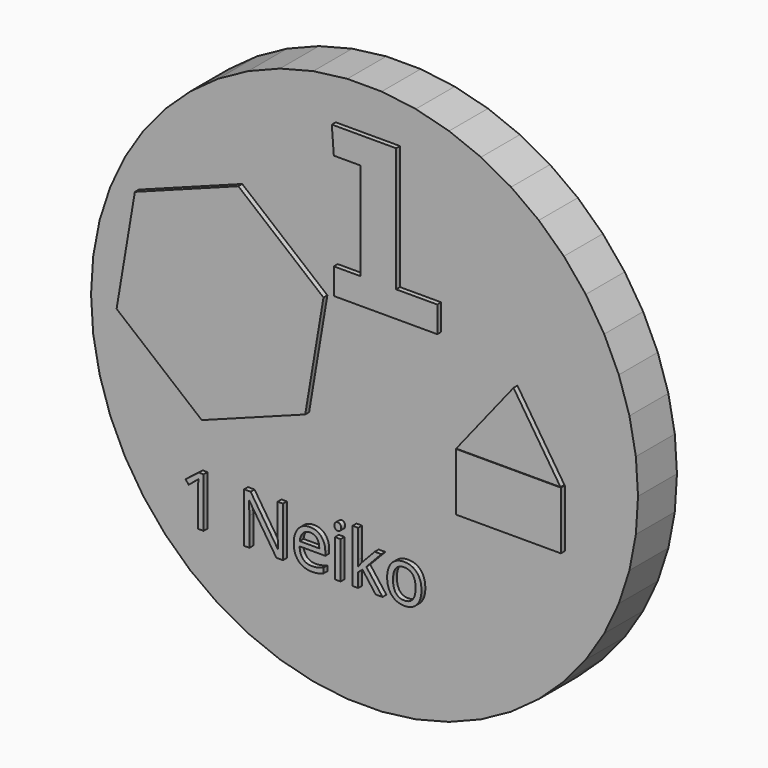
from build123d import *

# Parameters (mm, degrees)
F1_DEPTH     = 10
F7_R         = 52.6569549138
F8_DEPTH     = 1
F9_R         = 17.4080178081
F10_DEPTH    = 1
F3_TEXT_SIZE = 14.3319963374
F11_DEPTH    = 1
F5_W         = 21.5642787516
F5_H         = 11.8847033009
F12_DEPTH    = 1


# Not quite as in the source:
# - Text() gives the source's letters only with a copy of the font that has no kerning and outlines rounded to 1/6400 em; it was checked with that copy


with BuildPart() as f1:
    # F0 (on Front) → F1 (new body)
    with BuildSketch(Plane.XZ):
        Polygon((3.5282940617, 56.0806281865), (-3.5282940617, 56.0806281865), (-10.5292388801, 55.196203179), (-17.3641313115, 53.4413010748), (-23.9251810193, 50.8435977284), (-30.1089163302, 47.4440604733), (-35.8178160444, 43.2963020428), (-40.961847403, 38.4657350652), (-45.4598859587, 33.0285404673), (-49.2409949564, 27.0704660559), (-52.2455440484, 20.6854742237), (-54.4261497009, 13.974260106), (-55.74842246, 7.0426635587), (-56.1915092943, 0), (-55.74842246, -7.0426635587), (-54.4261497009, -13.974260106), (-52.2455440484, -20.6854742237), (-49.2409949564, -27.0704660559), (-45.4598859587, -33.0285404673), (-40.961847403, -38.4657350652), (-35.8178160444, -43.2963020428), (-30.1089163302, -47.4440604733), (-23.9251810193, -50.8435977284), (-17.3641313115, -53.4413010748), (-10.5292388801, -55.196203179), (-3.5282940617, -56.0806281865), (3.5282940617, -56.0806281865), (10.5292388801, -55.196203179), (17.3641313115, -53.4413010748), (23.9251810193, -50.8435977284), (30.1089163302, -47.4440604733), (35.8178160444, -43.2963020428), (40.961847403, -38.4657350652), (45.4598859587, -33.0285404673), (49.2409949564, -27.0704660559), (52.2455440484, -20.6854742237), (54.4261497009, -13.974260106), (55.74842246, -7.0426635587), (56.1915092943, 0), (55.74842246, 7.0426635587), (54.4261497009, 13.974260106), (52.2455440484, 20.6854742237), (49.2409949564, 27.0704660559), (45.4598859587, 33.0285404673), (40.961847403, 38.4657350652), (35.8178160444, 43.2963020428), (30.1089163302, 47.4440604733), (23.9251810193, 50.8435977284), (17.3641313115, 53.4413010748), (10.5292388801, 55.196203179), align=None)
    extrude(amount=F1_DEPTH)

    # F7 (on face) → F8 (join)
    with BuildSketch(Plane(origin=(0, 0, 0), x_dir=(-1, 0, 0), z_dir=(0, 1, 0))):
        Circle(F7_R)
    extrude(amount=F8_DEPTH)

    # F9 (on face) → F10 (join)
    with BuildSketch(Plane(origin=(0, 1, 0), x_dir=(-1, 0, 0), z_dir=(0, 1, 0))):
        Circle(F9_R)
    extrude(amount=F10_DEPTH)

    # F2 (on face) + F6 (on face) + F4 (on face) + F3 (on face) → F11 (join)
    with BuildSketch(Plane.XZ.offset(10)):
        Polygon((7.2863269597, 47.4440604733), (-5.9220409021, 47.4440604733), (-5.5092796683, 41.951071471), (0, 41.951071471), (0, 21.9321399927), (-5.5092796683, 21.9321399927), (-5.5092796683, 16.5662392974), (15.7479383051, 16.5662392974), (15.7479383051, 21.9321399927), (7.2863269597, 21.9321399927), align=None)
    with BuildSketch(Plane.XZ.offset(10)):
        Polygon((31.4109884202, 11.9623439386), (19.6289718151, -2.851766767), (41.0649701953, -2.851766767), align=None)
    with BuildSketch(Plane.XZ.offset(10)):
        Polygon((-25.1322471832, 30.0395505261), (-46.3870606089, 22.1044181157), (-50.142441072, -0.2703564688), (-32.6430081094, -14.709998643), (-11.3881946837, -6.7748662327), (-7.6328142206, 15.5999083519), align=None)
    with BuildSketch(Plane.XZ.offset(10)):
        with Locations((-37.2696332633, -34.6274599433)):
            Text('1 Neiko', F3_TEXT_SIZE, font='Open Sans', text_align=(TextAlign.LEFT, TextAlign.BOTTOM))
    extrude(amount=F11_DEPTH)

    # F5 (on face) → F12 (join)
    with BuildSketch(Plane.XZ.offset(10)):
        with Locations((30.3556639701, -8.8731837459)):
            Rectangle(F5_W, F5_H)
    extrude(amount=F12_DEPTH)

    # F13 (on face) → F14 (revolve)
    with BuildSketch(Plane(origin=(0, 2, 0), x_dir=(-1, 0, 0), z_dir=(0, 1, 0))):
        with BuildLine():
            Line((0, 7.3307841085), (0, -8.7448451668))
            ThreePointArc((0, -8.7448451668), (7.4222381642, -0.7070305292), (0, 7.3307841085))
        make_face()
    revolve(axis=Axis((0, 2, -0.7070305292), (0, 0, -1)))


solid = f1.part
